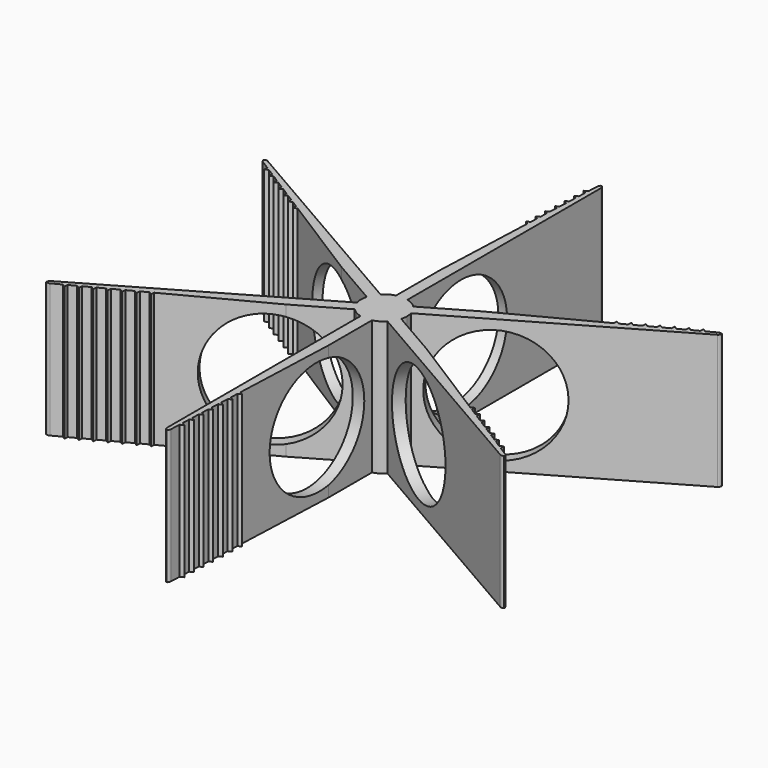
from build123d import *

# Parameters (mm, degrees)
F1_DEPTH    = 35
F2_T1_DEPTH = 294.9923167973
F3_T1_DEPTH = 40
F3_T3_DEPTH = 39.8039984013
F4_R        = 15
F5_DEPTH    = 3.001
F7_DEPTH    = 35
F8_COUNT    = 6


# Not quite as in the source:
# - a fillet or chamfer that OpenCascade refuses, or shapes differently, is made with other operations: its cross-section is extruded or revolved along the edge and cut away or added
# - ends of sketch curves that miss each other by under 0.0002 mm in the source are joined


with BuildPart() as f1:
    # F0 (on Top) → F1 (new body)
    with BuildSketch(Plane.XY):
        with BuildLine():
            Line((1.5, 70), (-1.5, 70))
            Line((-1.5, 70), (-1.5, 5.8094750193))
            ThreePointArc((-1.5, 5.8094750193), (0, 6), (1.5, 5.8094750193))
            Line((1.5, 5.8094750193), (1.5, 70))
        make_face()
        with BuildLine():
            ThreePointArc((1.5, 5.8094750193), (0, 6), (-1.5, 5.8094750193))
            Line((-1.5, 5.8094750193), (-1.5, 0))
            Line((-1.5, 0), (1.5, 0))
            Line((1.5, 0), (1.5, 5.8094750193))
        make_face()
        with BuildLine():
            Line((-1.5, 0), (-1.5, 5.8094750193))
            ThreePointArc((-1.5, 5.8094750193), (-3.6742346142, -4.7434164903), (6, 0))
            ThreePointArc((6, 0), (4.7434164903, 3.6742346142), (1.5, 5.8094750193))
            Line((1.5, 5.8094750193), (1.5, 0))
            Line((1.5, 0), (-1.5, 0))
        make_face()
    extrude(amount=F1_DEPTH)

    # F2: chamfer of 2 x 50 on 1 edges, made by hand

    # F2_s2 → F2_t1 (cut)
    with BuildSketch(Plane.XY.offset(-129.9961583986)):
        Polygon((0.5, 70), (-1.5, 20), (-1.5, 70), align=None)
    extrude(amount=F2_T1_DEPTH, mode=Mode.SUBTRACT)

    # F3: fillet of radius 1 on 2 edges, made by hand

    # F3_s2 → F3_t1 (cut)
    with BuildSketch(Plane.XY.offset(-2.5)):
        with BuildLine():
            ThreePointArc((0.5, 70), (1.2071067812, 69.7071067812), (1.5, 69))
            Line((1.5, 69), (1.5, 70))
            Line((1.5, 70), (0.5, 70))
        make_face()
    extrude(amount=F3_T1_DEPTH, mode=Mode.SUBTRACT)

    # F3_s4 → F3_t3 (cut)
    with BuildSketch(Plane.XY.offset(-2.4019992006)):
        with BuildLine():
            ThreePointArc((1.4607996803, 70), (0.7679678242, 69.7210991743), (0.4615987215, 69.0399680383))
            Line((0.4615987215, 69.0399680383), (0.5, 70))
            Line((0.5, 70), (1.4607996803, 70))
        make_face()
    extrude(amount=F3_T3_DEPTH, mode=Mode.SUBTRACT)

    # F4 (on face) → F5 (cut, through all)
    with BuildSketch(Plane.YZ.offset(1.5)):
        with Locations((23.3094750193, 17.5)):
            Circle(F4_R)
    extrude(amount=-F5_DEPTH, mode=Mode.SUBTRACT)

    # F6 (on face) → F7 (join)
    with BuildSketch(Plane.XY.offset(35)):
        Polygon((-1.2504768379, 47.8892910339), (-0.4058017057, 47.3549573582), (-0.3658219397, 48.3544515083), align=None)
        Polygon((-1.1306456583, 50.8868968266), (-0.2858992768, 50.3525180794), (-0.2459161385, 51.3520965377), align=None)
        Polygon((-0.165996848, 53.3500788005), (-0.1260103373, 54.3497415672), (-1.0108144786, 53.8845026193), align=None)
        Polygon((-0.0460944191, 56.3476395216), (-0.0061045361, 57.3473865966), (-0.890983299, 56.8821084119), align=None)
        Polygon((0.0738080097, 59.3452002427), (0.113801265, 60.345031626), (-0.7711521193, 59.8797142046), align=None)
        Polygon((0.1937087524, 62.3427188097), (0.2337087524, 63.3427188097), (-0.6513209396, 62.8773199973), align=None)
        Polygon((0.3136128674, 65.3403216849), (0.3536128674, 66.3403216849), (-0.53148976, 65.87492579), align=None)
    extrude(amount=-F7_DEPTH)

    # F8: F1 ×6 about axis
    f8_axis = Axis((0, 0, 0), (0, 0, -1))


with BuildPart() as f1_1:
    add(f1.part)
    for i in range(1, F8_COUNT):
        add(f1.part.rotate(f8_axis, i * 360 / F8_COUNT))


solid = f1_1.part
